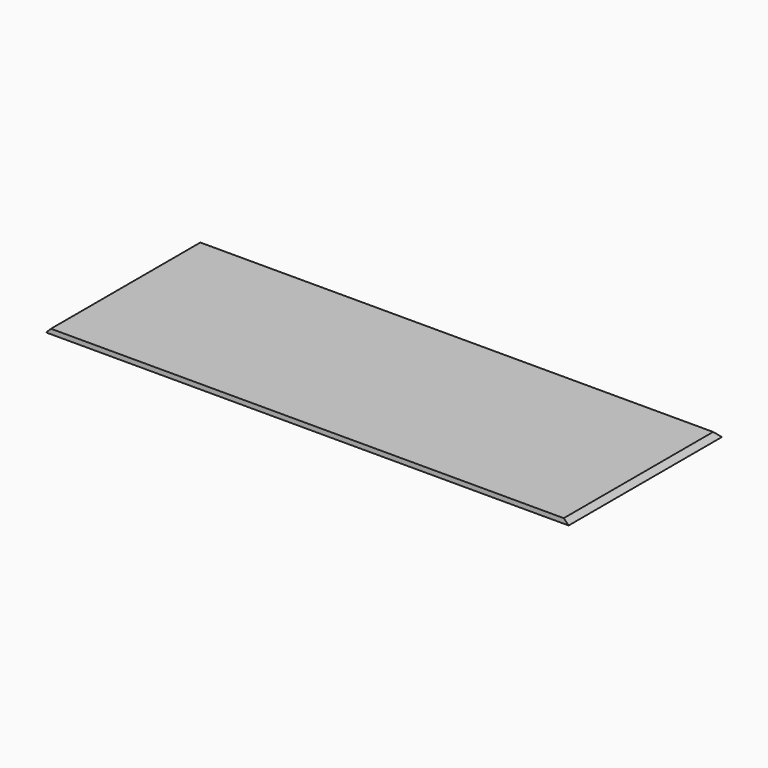
from build123d import *

# Parameters (mm, degrees)
F0_W     = 1500
F0_H     = 550
F1_DEPTH = 14
F2_SIZE  = 13.99999


# Not quite as in the source:
# - a fillet or chamfer is up to 0.001 mm smaller than in the source, because OpenCascade refuses the exact size


with BuildPart() as f1:
    # F0 (on Top) → F1 (new body)
    with BuildSketch(Plane.XY):
        Rectangle(F0_W, F0_H)
    extrude(amount=F1_DEPTH)

    # F2 (size 14 in the source; OpenCascade refuses exactly that, so slightly less here)
    f2_edges = [f1.edges().sort_by_distance(p)[0] for p in [
        (-750, 0, 14),
        (0, 275, 14),
        (750, 0, 14),
    ]]
    chamfer(f2_edges, length=F2_SIZE)


solid = f1.part
